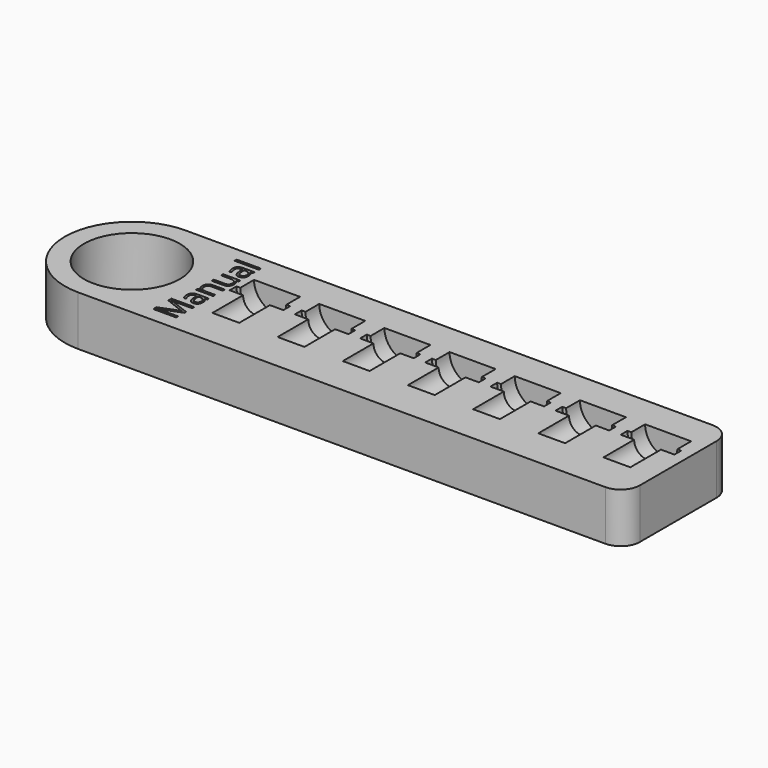
from build123d import *

# Parameters (mm, degrees)
F0_R          = 12.5
F1_DEPTH      = 13
F10_TEXT_SIZE = 8.3468249685
F11_DEPTH     = 2
F19_TEXT_SIZE = 9.0855688271
F20_DEPTH     = 2


# Not quite as in the source:
# - Text() gives the source's letters only with a copy of the font that has no kerning and outlines rounded to 1/6400 em; it was checked with that copy


with BuildPart() as f1:
    # F0 (on Top) → F1 (new body)
    with BuildSketch(Plane.XY):
        with BuildLine():
            ThreePointArc((0, 17.5), (5.1256313292, 5.1256313292), (17.5, 0))
            Line((17.5, 0), (155, 0))
            ThreePointArc((155, 0), (158.5355339059, 1.4644660941), (160, 5))
            Line((160, 5), (160, 30))
            ThreePointArc((160, 30), (158.5355339059, 33.5355339059), (155, 35))
            Line((155, 35), (17.5, 35))
            ThreePointArc((17.5, 35), (5.1256313292, 29.8743686708), (0, 17.5))
        make_face()
        with Locations((17.5, 17.5)):
            Circle(F0_R, mode=Mode.SUBTRACT)
    extrude(amount=F1_DEPTH)

    # F2 (on face) → F3 (revolve, cut)
    with BuildSketch(Plane.XY.offset(13)):
        Polygon((48, 20), (48, 10), (51.5, 10), (51.5, 20), (55, 20), (55, 22.2), (54, 22.2), (54, 26.7), (48, 26.7), (48, 22.2), align=None)
    revolve(axis=Axis((48, 15, 13), (0, 1, 0)), mode=Mode.SUBTRACT)

    # F2 (on face) → F4 (revolve, cut)
    with BuildSketch(Plane.XY.offset(13)):
        Polygon((65, 20), (65, 10), (68.5, 10), (68.5, 20), (72, 20), (72, 22.2), (71, 22.2), (71, 26.7), (65, 26.7), (65, 22.2), align=None)
    revolve(axis=Axis((65, 15, 13), (0, 1, 0)), mode=Mode.SUBTRACT)

    # F2 (on face) → F5 (revolve, cut)
    with BuildSketch(Plane.XY.offset(13)):
        Polygon((82, 20), (82, 10), (85.5, 10), (85.5, 20), (89, 20), (89, 22.2), (88, 22.2), (88, 26.7), (82, 26.7), (82, 22.2), align=None)
    revolve(axis=Axis((82, 15, 13), (0, 1, 0)), mode=Mode.SUBTRACT)

    # F2 (on face) → F6 (revolve, cut)
    with BuildSketch(Plane.XY.offset(13)):
        Polygon((99, 20), (99, 10), (102.5, 10), (102.5, 20), (106, 20), (106, 22.2), (105, 22.2), (105, 26.7), (99, 26.7), (99, 22.2), align=None)
    revolve(axis=Axis((99, 15, 13), (0, 1, 0)), mode=Mode.SUBTRACT)

    # F2 (on face) → F7 (revolve, cut)
    with BuildSketch(Plane.XY.offset(13)):
        Polygon((116, 20), (116, 10), (119.5, 10), (119.5, 20), (123, 20), (123, 22.2), (122, 22.2), (122, 26.7), (116, 26.7), (116, 22.2), align=None)
    revolve(axis=Axis((116, 15, 13), (0, 1, 0)), mode=Mode.SUBTRACT)

    # F2 (on face) → F8 (revolve, cut)
    with BuildSketch(Plane.XY.offset(13)):
        Polygon((133, 20), (133, 10), (136.5, 10), (136.5, 20), (140, 20), (140, 22.2), (139, 22.2), (139, 26.7), (133, 26.7), (133, 22.2), align=None)
    revolve(axis=Axis((133, 15, 13), (0, 1, 0)), mode=Mode.SUBTRACT)

    # F2 (on face) → F9 (revolve, cut)
    with BuildSketch(Plane.XY.offset(13)):
        Polygon((150, 20), (150, 10), (153.5, 10), (153.5, 20), (157, 20), (157, 22.2), (156, 22.2), (156, 26.7), (150, 26.7), (150, 22.2), align=None)
    revolve(axis=Axis((150, 15, 13), (0, 1, 0)), mode=Mode.SUBTRACT)

    # F10 (on face) → F11 (cut)
    with BuildSketch(Plane.XY.offset(13)):
        with Locations(Location((40, 3), (0, 0, 90))):
            Text('Manual', F10_TEXT_SIZE, font='Open Sans', text_align=(TextAlign.LEFT, TextAlign.BOTTOM))
    extrude(amount=-F11_DEPTH, mode=Mode.SUBTRACT)

    # F12 (on face) → F13 (revolve, cut)
    with BuildSketch(Plane(origin=(0, 0, 0), x_dir=(1, 0, 0), z_dir=(0, 0, -1))):
        Polygon((65, -15), (65, -25), (69, -25), (69, -15), (72.5, -15), (72.5, -12.8), (71.5, -12.8), (71.5, -8.3), (65, -8.3), (65, -12.8), align=None)
    revolve(axis=Axis((65, 20, 0), (0, -1, 0)), mode=Mode.SUBTRACT)

    # F12 (on face) → F14 (revolve, cut)
    with BuildSketch(Plane(origin=(0, 0, 0), x_dir=(1, 0, 0), z_dir=(0, 0, -1))):
        Polygon((82, -15), (82, -25), (86, -25), (86, -15), (89.5, -15), (89.5, -12.8), (88.5, -12.8), (88.5, -8.3), (82, -8.3), (82, -12.8), align=None)
    revolve(axis=Axis((82, 20, 0), (0, -1, 0)), mode=Mode.SUBTRACT)

    # F12 (on face) → F15 (revolve, cut)
    with BuildSketch(Plane(origin=(0, 0, 0), x_dir=(1, 0, 0), z_dir=(0, 0, -1))):
        Polygon((99, -15), (99, -25), (103, -25), (103, -15), (106.5, -15), (106.5, -12.8), (105.5, -12.8), (105.5, -8.3), (99, -8.3), (99, -12.8), align=None)
    revolve(axis=Axis((99, 20, 0), (0, -1, 0)), mode=Mode.SUBTRACT)

    # F12 (on face) → F16 (revolve, cut)
    with BuildSketch(Plane(origin=(0, 0, 0), x_dir=(1, 0, 0), z_dir=(0, 0, -1))):
        Polygon((116, -15), (116, -25), (120, -25), (120, -15), (123.5, -15), (123.5, -12.8), (122.5, -12.8), (122.5, -8.3), (116, -8.3), (116, -12.8), align=None)
    revolve(axis=Axis((116, 20, 0), (0, -1, 0)), mode=Mode.SUBTRACT)

    # F12 (on face) → F17 (revolve, cut)
    with BuildSketch(Plane(origin=(0, 0, 0), x_dir=(1, 0, 0), z_dir=(0, 0, -1))):
        Polygon((133, -15), (133, -25), (137, -25), (137, -15), (140.5, -15), (140.5, -12.8), (139.5, -12.8), (139.5, -8.3), (133, -8.3), (133, -12.8), align=None)
    revolve(axis=Axis((133, 20, 0), (0, -1, 0)), mode=Mode.SUBTRACT)

    # F12 (on face) → F18 (revolve, cut)
    with BuildSketch(Plane(origin=(0, 0, 0), x_dir=(1, 0, 0), z_dir=(0, 0, -1))):
        Polygon((150, -15), (150, -25), (154, -25), (154, -15), (157.5, -15), (157.5, -12.8), (156.5, -12.8), (156.5, -8.3), (150, -8.3), (150, -12.8), align=None)
    revolve(axis=Axis((150, 20, 0), (0, -1, 0)), mode=Mode.SUBTRACT)

    # F19 (on face) → F20 (cut)
    with BuildSketch(Plane(origin=(0, 0, 0), x_dir=(1, 0, 0), z_dir=(0, 0, -1))):
        with Locations(Location((40, -32), (0, 0, 90))):
            Text('Power', F19_TEXT_SIZE, font='Open Sans', font_style=FontStyle.BOLD, text_align=(TextAlign.LEFT, TextAlign.BOTTOM))
    extrude(amount=-F20_DEPTH, mode=Mode.SUBTRACT)


solid = f1.part
